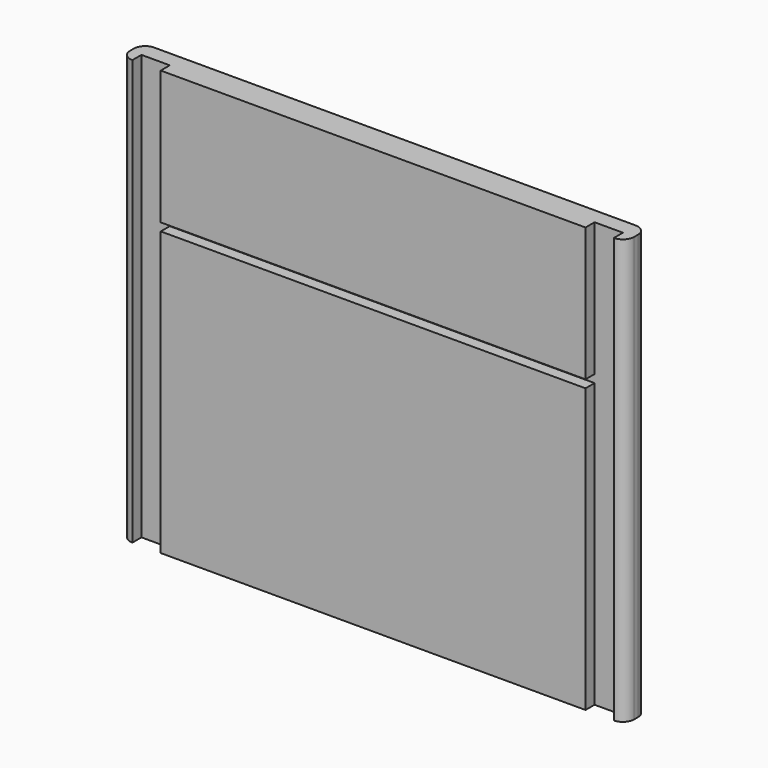
from build123d import *

# Parameters (mm, degrees)
F0_W     = 89
F0_H     = 75
F1_DEPTH = 4.8
F2_W     = 75
F2_H     = 1.4
F3_DEPTH = 2
F4_R     = 1.99999


# Not quite as in the source:
# - a fillet or chamfer is up to 0.001 mm smaller than in the source, because OpenCascade refuses the exact size


with BuildPart() as f1:
    # F0 (on Front) → F1 (new body)
    with BuildSketch(Plane.XZ):
        Rectangle(F0_W, F0_H)
    extrude(amount=F1_DEPTH)

    # F2 (on face) → F3 (cut)
    with BuildSketch(Plane.XZ.offset(4.8)):
        Polygon((-42.5, 37.5), (-42.5, -37.5), (-37.5, -37.5), (-37.5, 12.5), (-37.5, 13.9), (-37.5, 37.5), align=None)
        with Locations((0, 13.2)):
            Rectangle(F2_W, F2_H)
        Polygon((37.5, 13.9), (37.5, 12.5), (37.5, -37.5), (42.5, -37.5), (42.5, 37.5), (37.5, 37.5), align=None)
    extrude(amount=-F3_DEPTH, mode=Mode.SUBTRACT)

    # F4 (radius 2 in the source; OpenCascade refuses exactly that, so slightly less here)
    f4_edges = [f1.edges().sort_by_distance(p)[0] for p in [
        (-44.5, -4.8, 0),
        (44.5, -4.8, 0),
        (44.5, 0, 0),
        (-44.5, 0, 0),
    ]]
    fillet(f4_edges, radius=F4_R)


solid = f1.part
